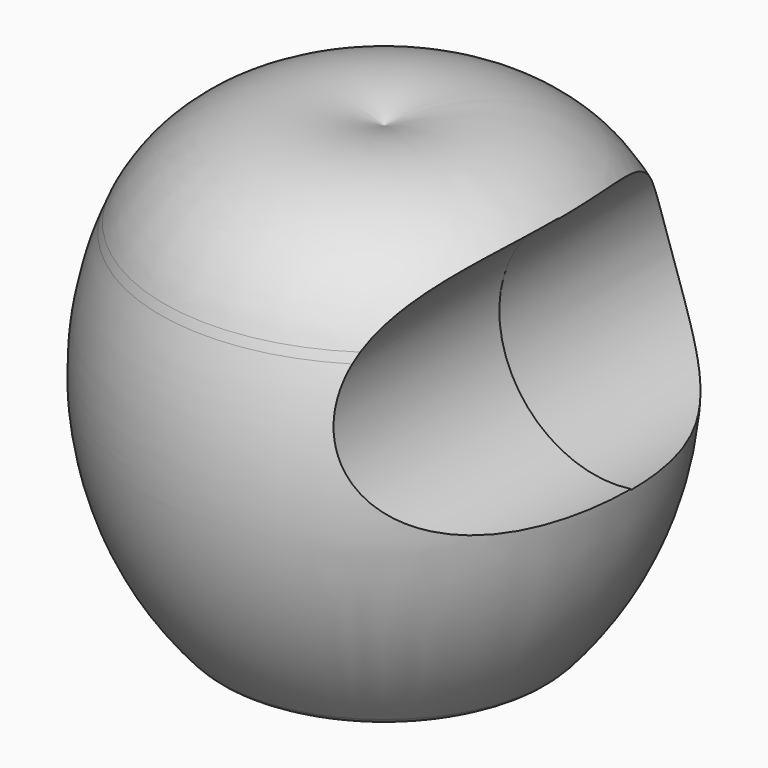
from build123d import *

# Parameters (mm, degrees)
F2_R     = 10.16
F3_DEPTH = 21.8131542984
F4_R     = 2.54
F5_R     = 10.16
F6_DEPTH = 21.8131542984


# Not quite as in the source:
# - a feature names something its author has since deleted; it is built from what else it names


with BuildPart() as f1:
    # F0 (on Front) → F1 (revolve)
    with BuildSketch(Plane.XZ):
        with BuildLine():
            ThreePointArc((-12.2520654017, -18.0816771193), (-6.7605609497, -13.8304712842), (0, -15.4192405701))
            Line((0, -15.4192405701), (0, 22.6807594299))
            ThreePointArc((0, 22.6807594299), (-11.239053287, 22.9003327562), (-19.3984057777, 15.1679658374))
            ThreePointArc((-19.3984057777, 15.1679658374), (-19.5624851514, 14.7821444157), (-19.7210129028, 14.394008921))
            ThreePointArc((-19.7210129028, 14.394008921), (-21.0686031127, -3.0126367804), (-12.2520654017, -18.0816771193))
        make_face()
    revolve(axis=Axis((0, 0, 3.6307594299), (0, 0, -1)))

    # F2 (on Front) → F3 (cut, through all)
    with BuildSketch(Plane.XZ):
        with Locations((20.2043764293, 11.5205561742)):
            Circle(F2_R)
    extrude(amount=-F3_DEPTH, mode=Mode.SUBTRACT)

    # F4
    f4_edges = [f1.edges().sort_by_distance(p)[0] for p in [
        (12.252065, 0, -18.081677),
    ]]
    fillet(f4_edges, radius=F4_R)

    # F5 (on Front) → F6 (cut, through all)
    with BuildSketch(Plane.XZ):
        with Locations((20.2997829765, 11.6159608588)):
            Circle(F5_R)
    extrude(amount=F6_DEPTH, mode=Mode.SUBTRACT)


solid = f1.part
